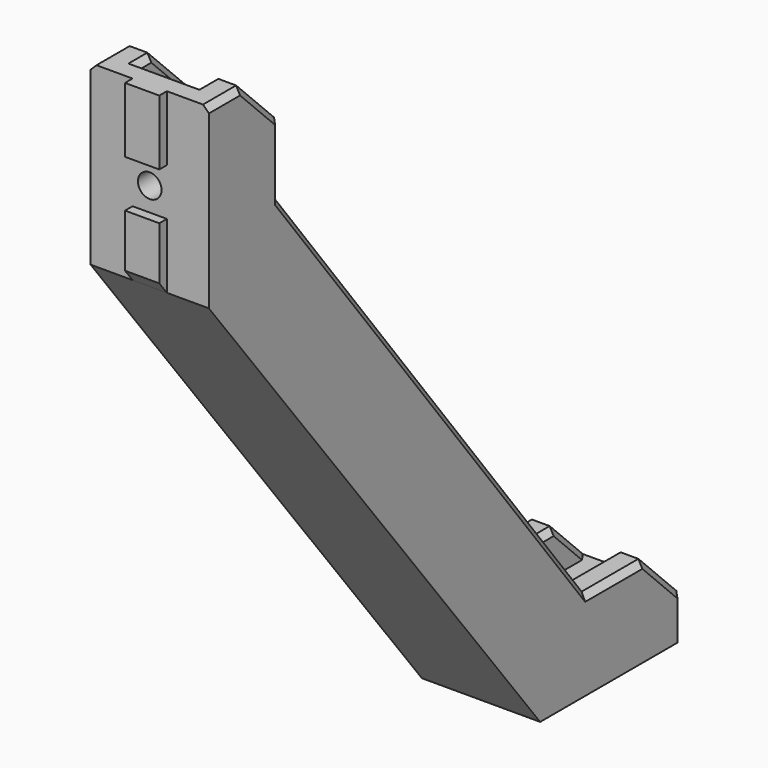
from build123d import *

# Parameters (mm, degrees)
F1_DEPTH    = 10
F2_W        = 5.8
F2_H        = 30
F3_DEPTH    = 1.6
F4_W        = 5.8
F4_H        = 8
F5_DEPTH    = 1.6
F6_R        = 2
F7_DEPTH    = 15
F9_DEPTH    = 5
F10_R       = 3.25
F11_DEPTH   = 8
F13_DEPTH   = 5.8
F14_C1_SIZE = 8
F14_C2_SIZE = 8
F14_C3_SIZE = 8
F15_SIZE    = 1


with BuildPart() as f1:
    # F0 (on Right) → F1 (new body, symmetric)
    with BuildSketch(Plane.YZ):
        Polygon((70, 0), (100, 0), (100, 15), (80, 15), (15, 100), (15, 120), (0, 120), (0, 90), align=None)
    extrude(amount=F1_DEPTH, both=True)

    # F2 (on face) → F3 (join)
    with BuildSketch(Plane.XZ):
        with Locations((0, 105)):
            Rectangle(F2_W, F2_H)
    extrude(amount=F3_DEPTH)

    # F4 (on face) → F5 (cut, through all)
    with BuildSketch(Plane.XZ.offset(1.6)):
        with Locations((0, 105)):
            Rectangle(F4_W, F4_H)
    extrude(amount=-F5_DEPTH, mode=Mode.SUBTRACT)

    # F6 (on face) → F7 (cut, through all)
    with BuildSketch(Plane.XZ):
        with Locations((0, 105)):
            Circle(F6_R)
    extrude(amount=-F7_DEPTH, mode=Mode.SUBTRACT)

    # F8 (on Right) → F9 (cut, symmetric)
    with BuildSketch(Plane.YZ):
        Polygon((21.8223074079, 120), (4, 120), (4, 100), (75.5555555556, 8), (100, 8), (100, 19.4858238101), align=None)
    extrude(amount=F9_DEPTH, both=True, mode=Mode.SUBTRACT)

    # F10 (on face) → F11 (cut, through all)
    with BuildSketch(Plane.XY.offset(8)):
        with Locations((0, 86)):
            Circle(F10_R)
    extrude(amount=-F11_DEPTH, mode=Mode.SUBTRACT)

    # F12 (on face) → F13 (cut, through all)
    with BuildSketch(Plane.YZ.offset(2.9)):
        Polygon((-1.6, 90), (0, 90), (-1.6, 92.0571428571), align=None)
    extrude(amount=-F13_DEPTH, mode=Mode.SUBTRACT)

    # F14: chamfer of 8 on 4 edges, made by hand

    # F14_c1
    f14_c1_edges = [f1.edges().sort_by_distance(p)[0] for p in [
        (7.5, 100, 15),
    ]]
    chamfer(f14_c1_edges, length=F14_C1_SIZE)

    # F14_c2
    f14_c2_edges = [f1.edges().sort_by_distance(p)[0] for p in [
        (-7.5, 15, 120),
    ]]
    chamfer(f14_c2_edges, length=F14_C2_SIZE)

    # F14_c3
    f14_c3_edges = [f1.edges().sort_by_distance(p)[0] for p in [
        (7.5, 15, 120),
    ]]
    chamfer(f14_c3_edges, length=F14_C3_SIZE)

    # F15
    f15_edges = [f1.edges().sort_by_distance(p)[0] for p in [
        (10, 47.5, 57.5),
        (5, 47.5, 57.5),
        (10, 15, 106),
        (5, 15, 106),
        (-5, 15, 106),
        (-10, 15, 106),
        (-5, 47.5, 57.5),
        (-10, 47.5, 57.5),
        (10, 86, 15),
        (5, 86, 15),
        (-5, 86, 15),
        (-10, 86, 15),
        (-10, 100, 3.5),
        (10, 100, 3.5),
        (10, 3.5, 120),
        (5, 5.5, 120),
        (-5, 5.5, 120),
        (-10, 3.5, 120),
        (0, 4, 120),
        (5, 39.777778, 54),
        (-5, 39.777778, 54),
        (10, 96, 11),
        (5, 95.5, 11.5),
        (-5, 95.5, 11.5),
        (-10, 96, 11),
        (10, 11, 116),
        (5, 11, 116),
        (-5, 11, 116),
        (-10, 11, 116),
    ]]
    chamfer(f15_edges, length=F15_SIZE)


solid = f1.part
